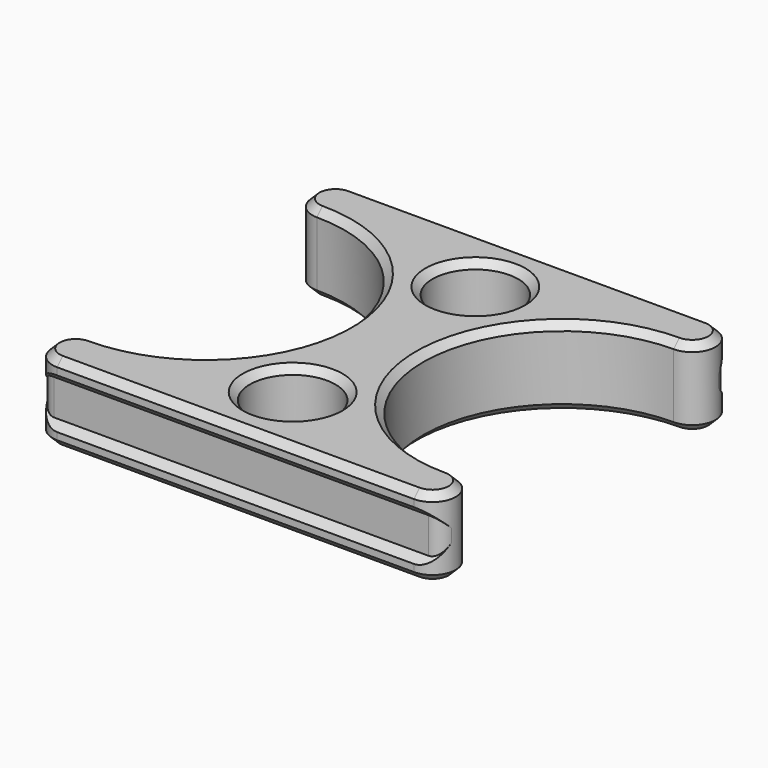
from build123d import *

# Parameters (mm, degrees)
F1_DEPTH  = 11
F2_W      = 9.2488363385
F2_H      = 7
F2_W_2    = 50
F3_DEPTH  = 1
F6_SIZE   = 1
F7_SIZE   = 0.99999
F8_R      = 2
F9_R      = 6
F10_DEPTH = 11.001
F11_SIZE  = 1


# Not quite as in the source:
# - a fillet or chamfer is up to 0.001 mm smaller than in the source, because OpenCascade refuses the exact size


with BuildPart() as f1:
    # F0 (on Top) → F1 (new body)
    with BuildSketch(Plane.XY):
        with BuildLine():
            ThreePointArc((-25, 19.5), (-5.5, 0), (-25, -19.5))
            ThreePointArc((-25, -19.5), (-28.25, -22.75), (-25, -26))
            Line((-25, -26), (25, -26))
            ThreePointArc((25, -26), (28.25, -22.75), (25, -19.5))
            ThreePointArc((25, -19.5), (5.5, 0), (25, 19.5))
            ThreePointArc((25, 19.5), (28.25, 22.75), (25, 26))
            Line((25, 26), (-25, 26))
            ThreePointArc((-25, 26), (-28.25, 22.75), (-25, 19.5))
        make_face()
        with BuildLine():
            ThreePointArc((-25, -24), (-26.25, -22.75), (-25, -21.5))
            ThreePointArc((-25, -21.5), (-3.5, 0), (-25, 21.5))
            ThreePointArc((-25, 21.5), (-26.25, 22.75), (-25, 24))
            Line((-25, 24), (25, 24))
            ThreePointArc((25, 24), (26.25, 22.75), (25, 21.5))
            ThreePointArc((25, 21.5), (3.5, 0), (25, -21.5))
            ThreePointArc((25, -21.5), (26.25, -22.75), (25, -24))
            Line((25, -24), (-25, -24))
        make_face(mode=Mode.SUBTRACT)
        with BuildLine():
            ThreePointArc((-25, 21.5), (-3.5, 0), (-25, -21.5))
            ThreePointArc((-25, -21.5), (-26.25, -22.75), (-25, -24))
            Line((-25, -24), (25, -24))
            ThreePointArc((25, -24), (26.25, -22.75), (25, -21.5))
            ThreePointArc((25, -21.5), (3.5, 0), (25, 21.5))
            ThreePointArc((25, 21.5), (26.25, 22.75), (25, 24))
            Line((25, 24), (-25, 24))
            ThreePointArc((-25, 24), (-26.25, 22.75), (-25, 21.5))
        make_face()
    extrude(amount=F1_DEPTH)


with BuildPart() as f3:
    # F2 (on face) → F3 (new body)
    with BuildSketch(Plane.XZ.offset(26)):
        with Locations((-29.6244181693, 5.5)):
            Rectangle(F2_W, F2_H)
        with Locations((0, 5.5)):
            Rectangle(F2_W_2, F2_H)
        with Locations((29.6244181693, 5.5)):
            Rectangle(F2_W, F2_H)
    extrude(amount=-F3_DEPTH)


with BuildPart() as f4_1:
    # F4: copy of F3
    add(f3.part.moved(Location((0, 51, 0))))


with BuildPart() as f1_1:
    add(f1.part)

    # F5: cut F4_1, F3
    add(f4_1.part, mode=Mode.SUBTRACT)
    add(f3.part, mode=Mode.SUBTRACT)

    # F6
    f6_edges = [f1_1.edges().sort_by_distance(p)[0] for p in [
        (-5.5, 0, 11),
        (-5.5, 0, 0),
    ]]
    chamfer(f6_edges, length=F6_SIZE)

    # F7 (size 1 in the source; OpenCascade refuses exactly that, so slightly less here)
    f7_edges = [f1_1.edges().sort_by_distance(p)[0] for p in [
        (0, -25, 9),
        (0, -25, 2),
        (0, 25, 9),
        (0, 25, 2),
    ]]
    chamfer(f7_edges, length=F7_SIZE)

    # F8
    f8_edges = [f1_1.edges().sort_by_distance(p)[0] for p in [
        (27.345208, 25, 5.5),
        (-27.345208, 25, 5.5),
        (-27.345208, -25, 5.5),
        (27.345208, -25, 5.5),
    ]]
    fillet(f8_edges, radius=F8_R)

    # F9 (on face) → F10 (cut, through all)
    with BuildSketch(Plane.XY.offset(11)):
        with Locations((0, -16)):
            Circle(F9_R)
        with Locations((0, 16)):
            Circle(F9_R)
    extrude(amount=-F10_DEPTH, mode=Mode.SUBTRACT)

    # F11
    f11_edges = [f1_1.edges().sort_by_distance(p)[0] for p in [
        (-6, 16, 11),
        (-6, -16, 11),
        (-6, -16, 0),
        (-6, 16, 0),
    ]]
    chamfer(f11_edges, length=F11_SIZE)


solid = f1_1.part
